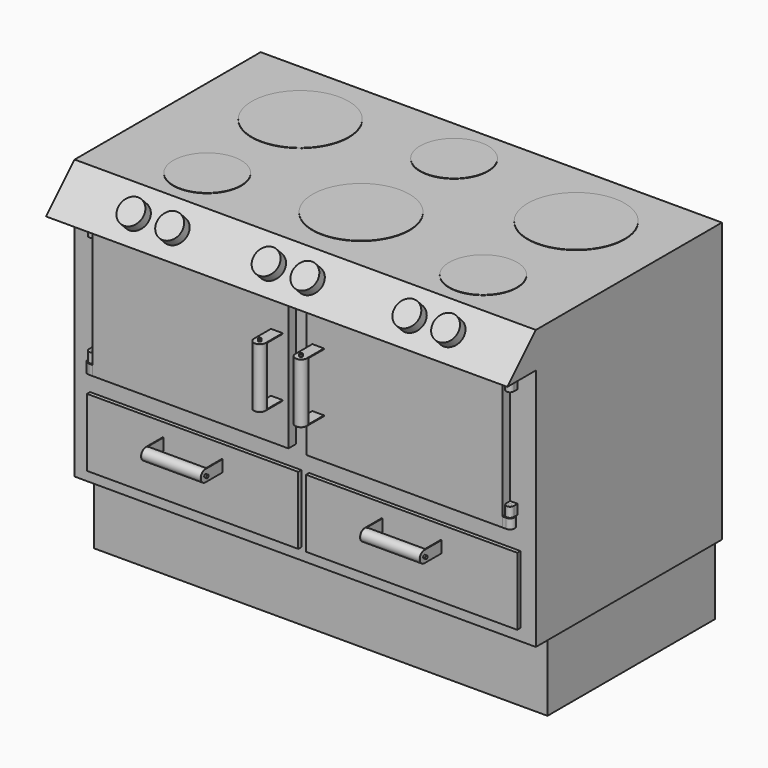
from build123d import *

# Parameters (mm, degrees)
F5_W           = 1190
F5_H           = 600
F6_DEPTH       = 720
F7_T           = -5
F8_W           = 465
F8_H           = 320
F9_DEPTH       = 25
F10_W          = 475
F10_H          = 330
F10_W_2        = 465
F10_H_2        = 320
F11_DEPTH      = 415
F12_W          = 475
F12_H          = 330
F13_DEPTH      = 5
F14_W          = 505
F14_H          = 150
F15_DEPTH      = 25
F16_W          = 515
F16_H          = 160
F16_W_2        = 505
F16_H_2        = 150
F17_DEPTH      = 470
F18_W          = 515
F18_H          = 160
F19_DEPTH      = 5
F20_R          = 6
F21_DEPTH      = 10
F22_R          = 6
F23_DEPTH      = 180
F25_DEPTH      = 10
F27_DEPTH      = 180
F28_W          = 505
F28_H          = 150
F29_DEPTH      = 475
F30_T          = -1
F30_2_T        = -1
F31_W          = 545
F31_H          = 175
F32_DEPTH      = 10
F33_W          = 505
F33_H          = 360
F34_DEPTH      = 25
F36_DEPTH      = 1190
F37_R          = 87.5
F38_DEPTH      = 1
F37_R_2        = 125
F39_R          = 4
F40_DEPTH      = 25
F41_R          = 4
F42_DEPTH      = 25
F43_R          = 4
F44_DEPTH      = 50
F49_R          = 45
F49_R_2        = 15
F50_DEPTH      = 25
F52_DEPTH      = 40
F54_R          = 4
F55_DEPTH      = 100
F56_W          = 475
F56_H          = 330
F56_W_2        = 471
F56_H_2        = 326
F57_DEPTH      = 80
F58_W          = 475
F58_H          = 330
F59_DEPTH      = 2
F60_W          = 475
F60_H          = 330
F61_DEPTH      = 502
F62_R          = 15
F62_R_2        = 4
F63_DEPTH      = 75
F64_R          = 4
F65_DEPTH      = 2
F67_R          = 4
F68_DEPTH      = 5
F68_DEPTH_BACK = 159
F71_R          = 15
F71_R_2        = 4
F72_DEPTH      = 75
F73_R          = 4
F74_DEPTH      = 2
F76_R          = 4
F77_DEPTH      = 5
F77_DEPTH_BACK = 159
F79_R          = 32.5
F80_DEPTH      = 25


with BuildPart() as f6:
    # F5 (on offset) → F6 (new body)
    with BuildSketch(Plane.XY.offset(190)):
        with Locations((595, -300)):
            Rectangle(F5_W, F5_H)
    extrude(amount=F6_DEPTH)

    # F7
    f7_openings = [f6.faces().sort_by_distance(p)[0] for p in [
        (595, 0, 550),
    ]]
    offset(amount=F7_T, openings=f7_openings)

    # F8 (on face) → F9 (cut)
    with BuildSketch(Plane.XZ.offset(600)):
        with Locations((870.8333333333, 630)):
            Rectangle(F8_W, F8_H)
        with Locations((319.1666666667, 630)):
            Rectangle(F8_W, F8_H)
    extrude(amount=-F9_DEPTH, mode=Mode.SUBTRACT)

    # F10 (on face) → F11 (join)
    with BuildSketch(Plane(origin=(0, -595, 0), x_dir=(-1, 0, 0), z_dir=(0, 1, 0))):
        with Locations((-870.8333333333, 630)):
            Rectangle(F10_W, F10_H)
        with Locations((-870.8333333333, 630)):
            Rectangle(F10_W_2, F10_H_2, mode=Mode.SUBTRACT)
        with Locations((-319.1666666667, 630)):
            Rectangle(F10_W, F10_H)
        with Locations((-319.1666666667, 630)):
            Rectangle(F10_W_2, F10_H_2, mode=Mode.SUBTRACT)
    extrude(amount=F11_DEPTH)

    # F12 (on face) → F13 (join)
    with BuildSketch(Plane(origin=(0, -180, 0), x_dir=(-1, 0, 0), z_dir=(0, 1, 0))):
        with Locations((-870.8333333333, 630)):
            Rectangle(F12_W, F12_H)
        with Locations((-319.1666666667, 630)):
            Rectangle(F12_W, F12_H)
    extrude(amount=F13_DEPTH)

    # F14 (on face) → F15 (cut)
    with BuildSketch(Plane.XZ.offset(600)):
        with Locations((312.5, 315)):
            Rectangle(F14_W, F14_H)
        with Locations((877.5, 315)):
            Rectangle(F14_W, F14_H)
    extrude(amount=-F15_DEPTH, mode=Mode.SUBTRACT)

    # F16 (on face) → F17 (join)
    with BuildSketch(Plane(origin=(0, -595, 0), x_dir=(-1, 0, 0), z_dir=(0, 1, 0))):
        with Locations((-877.5, 315)):
            Rectangle(F16_W, F16_H)
        with Locations((-877.5, 315)):
            Rectangle(F16_W_2, F16_H_2, mode=Mode.SUBTRACT)
        with Locations((-312.5, 315)):
            Rectangle(F16_W, F16_H)
        with Locations((-312.5, 315)):
            Rectangle(F16_W_2, F16_H_2, mode=Mode.SUBTRACT)
    extrude(amount=F17_DEPTH)

    # F18 (on face) → F19 (join)
    with BuildSketch(Plane(origin=(0, -125, 0), x_dir=(-1, 0, 0), z_dir=(0, 1, 0))):
        with Locations((-877.5, 315)):
            Rectangle(F18_W, F18_H)
        with Locations((-312.5, 315)):
            Rectangle(F18_W, F18_H)
    extrude(amount=F19_DEPTH)

    # F35 (on face) → F36 (join, through all)
    with BuildSketch(Plane(origin=(0, 0, 0), x_dir=(0, -1, 0), z_dir=(-1, 0, 0))):
        Polygon((691.9238815543, 818.0761184457), (600, 910), (600, 818.0761184457), align=None)
    extrude(amount=-F36_DEPTH)

    # F49 (on face) → F50 (cut)
    with BuildSketch(Plane(origin=(0, -175, 0), x_dir=(-1, 0, 0), z_dir=(0, 1, 0))):
        with Locations((-870.8333333333, 630)):
            Circle(F49_R)
        with Locations((-1058.3333333333, 745)):
            Circle(F49_R_2)
        with Locations((-1058.3333333333, 630)):
            Circle(F49_R_2)
        with Locations((-1058.3333333333, 515)):
            Circle(F49_R_2)
        with Locations((-691.8123364449, 745)):
            Circle(F49_R_2)
        with Locations((-691.8123364449, 630)):
            Circle(F49_R_2)
        with Locations((-683.3333333333, 515)):
            Circle(F49_R_2)
        with Locations((-319.1666666667, 630)):
            Circle(F49_R)
        with Locations((-506.6666666667, 745)):
            Circle(F49_R_2)
        with Locations((-506.6666666667, 630)):
            Circle(F49_R_2)
        with Locations((-506.6666666667, 515)):
            Circle(F49_R_2)
        with Locations((-131.6666666667, 630)):
            Circle(F49_R_2)
        with Locations((-131.6666666667, 745)):
            Circle(F49_R_2)
        with Locations((-131.6666666667, 515)):
            Circle(F49_R_2)
        with Locations((-319.1666666667, 515)):
            Circle(F49_R_2)
        with Locations((-319.1666666667, 745)):
            Circle(F49_R_2)
        with Locations((-870.8333333333, 745)):
            Circle(F49_R_2)
        with Locations((-870.8333333333, 515)):
            Circle(F49_R_2)
    extrude(amount=-F50_DEPTH, mode=Mode.SUBTRACT)


with BuildPart() as f21:
    # F20 (on face) → F21 (new body)
    with BuildSketch(Plane(origin=(0, 0, 190), x_dir=(1, 0, 0), z_dir=(0, 0, -1))):
        Polygon((44.5151724427, 490.5), (55.4848275573, 490.5), (60.9696551146, 500), (55.4848275573, 509.5), (44.5151724427, 509.5), (39.0303448854, 500), align=None)
        with Locations((50, 500)):
            Circle(F20_R, mode=Mode.SUBTRACT)
    extrude(amount=F21_DEPTH)


with BuildPart() as f21b:
    # F20 (on face) → F21, piece 2 (new body)
    with BuildSketch(Plane(origin=(0, 0, 190), x_dir=(1, 0, 0), z_dir=(0, 0, -1))):
        Polygon((1134.5151724427, 490.5), (1145.4848275573, 490.5), (1150.9696551146, 500), (1145.4848275573, 509.5), (1134.5151724427, 509.5), (1129.0303448854, 500), align=None)
        with Locations((1140, 500)):
            Circle(F20_R, mode=Mode.SUBTRACT)
    extrude(amount=F21_DEPTH)


with BuildPart() as f21c:
    # F20 (on face) → F21, piece 3 (new body)
    with BuildSketch(Plane(origin=(0, 0, 190), x_dir=(1, 0, 0), z_dir=(0, 0, -1))):
        Polygon((1145.4848275573, 40.5), (1150.9696551146, 50), (1145.4848275573, 59.5), (1134.5151724427, 59.5), (1129.0303448854, 50), (1134.5151724427, 40.5), align=None)
        with Locations((1140, 50)):
            Circle(F20_R, mode=Mode.SUBTRACT)
    extrude(amount=F21_DEPTH)


with BuildPart() as f21d:
    # F20 (on face) → F21, piece 4 (new body)
    with BuildSketch(Plane(origin=(0, 0, 190), x_dir=(1, 0, 0), z_dir=(0, 0, -1))):
        Polygon((40.0368294952, 45.4099491479), (48.9935153902, 39.0766158145), (58.956685895, 43.6666666667), (59.9631705048, 54.5900508521), (51.0064846098, 60.9233841855), (41.043314105, 56.3333333333), align=None)
        with Locations((50, 50)):
            Circle(F20_R, mode=Mode.SUBTRACT)
    extrude(amount=F21_DEPTH)


with BuildPart() as f23:
    # F22 (on face) → F23 (new body)
    with BuildSketch(Plane(origin=(0, 0, 190), x_dir=(1, 0, 0), z_dir=(0, 0, -1))):
        with Locations((50, 500)):
            Circle(F22_R)
    extrude(amount=F23_DEPTH)

    # F24 (on face) → F25, piece 4 (join)
    with BuildSketch(Plane(origin=(0, 0, 10), x_dir=(1, 0, 0), z_dir=(0, 0, -1))):
        Polygon((44.5151724427, 490.5), (55.4848275573, 490.5), (60.9696551146, 500), (55.4848275573, 509.5), (44.5151724427, 509.5), (39.0303448854, 500), align=None)
    extrude(amount=F25_DEPTH)


with BuildPart() as f23b:
    # F22 (on face) → F23, piece 2 (new body)
    with BuildSketch(Plane(origin=(0, 0, 190), x_dir=(1, 0, 0), z_dir=(0, 0, -1))):
        with Locations((50, 50)):
            Circle(F22_R)
    extrude(amount=F23_DEPTH)

    # F24 (on face) → F25, piece 3 (join)
    with BuildSketch(Plane(origin=(0, 0, 10), x_dir=(1, 0, 0), z_dir=(0, 0, -1))):
        Polygon((59.5, 44.5151724427), (59.5, 55.4848275573), (50, 60.9696551146), (40.5, 55.4848275573), (40.5, 44.5151724427), (50, 39.0303448854), align=None)
    extrude(amount=F25_DEPTH)


with BuildPart() as f23c:
    # F22 (on face) → F23, piece 3 (new body)
    with BuildSketch(Plane(origin=(0, 0, 190), x_dir=(1, 0, 0), z_dir=(0, 0, -1))):
        with Locations((1140, 50)):
            Circle(F22_R)
    extrude(amount=F23_DEPTH)

    # F24 (on face) → F25, piece 2 (join)
    with BuildSketch(Plane(origin=(0, 0, 10), x_dir=(1, 0, 0), z_dir=(0, 0, -1))):
        Polygon((1150.278965993, 53.830951768), (1141.8217814447, 60.8173215585), (1131.5428154518, 56.9863697906), (1129.721034007, 46.169048232), (1138.1782185553, 39.1826784415), (1148.4571845482, 43.0136302094), align=None)
    extrude(amount=F25_DEPTH)


with BuildPart() as f23d:
    # F22 (on face) → F23, piece 4 (new body)
    with BuildSketch(Plane(origin=(0, 0, 190), x_dir=(1, 0, 0), z_dir=(0, 0, -1))):
        with Locations((1140, 500)):
            Circle(F22_R)
    extrude(amount=F23_DEPTH)

    # F24 (on face) → F25 (join)
    with BuildSketch(Plane(origin=(0, 0, 10), x_dir=(1, 0, 0), z_dir=(0, 0, -1))):
        Polygon((1141.8217814447, 489.1826784415), (1150.278965993, 496.169048232), (1148.4571845482, 506.9863697906), (1138.1782185553, 510.8173215585), (1129.721034007, 503.830951768), (1131.5428154518, 493.0136302094), align=None)
    extrude(amount=F25_DEPTH)


with BuildPart() as f27:
    # F26 (on face) → F27 (new body)
    with BuildSketch(Plane(origin=(0, 0, 190), x_dir=(1, 0, 0), z_dir=(0, 0, -1))):
        Polygon((10, 550), (10, 10), (11, 10), (11, 549), (1179, 549), (1179, 10), (1180, 10), (1180, 550), align=None)
    extrude(amount=F27_DEPTH)


with BuildPart() as f29:
    # F28 (on face) → F29 (new body, through all)
    with BuildSketch(Plane.XZ.offset(125)):
        with Locations((312.5, 315)):
            Rectangle(F28_W, F28_H)
    extrude(amount=F29_DEPTH)

    # F30
    f30_openings = [f29.faces().sort_by_distance(p)[0] for p in [
        (312.5, -362.5, 390),
    ]]
    offset(amount=F30_T, openings=f30_openings)

    # F31 (on face) → F32 (join)
    with BuildSketch(Plane.XZ.offset(600)):
        with Locations((312.5, 307.5)):
            Rectangle(F31_W, F31_H)
    extrude(amount=F32_DEPTH)


with BuildPart() as f29b:
    # F28 (on face) → F29, piece 2 (new body, through all)
    with BuildSketch(Plane.XZ.offset(125)):
        with Locations((877.5, 315)):
            Rectangle(F28_W, F28_H)
    extrude(amount=F29_DEPTH)

    # F30#2
    f30_2_openings = [f29b.faces().sort_by_distance(p)[0] for p in [
        (877.5, -362.5, 390),
    ]]
    offset(amount=F30_2_T, openings=f30_2_openings)

    # F31 (on face) → F32, piece 2 (join)
    with BuildSketch(Plane.XZ.offset(600)):
        with Locations((877.5, 307.5)):
            Rectangle(F31_W, F31_H)
    extrude(amount=F32_DEPTH)


with BuildPart() as f34:
    # F33 (on face) → F34 (new body)
    with BuildSketch(Plane.XZ.offset(600)):
        with Locations((319.1666666667, 630)):
            Rectangle(F33_W, F33_H)
    extrude(amount=F34_DEPTH)


with BuildPart() as f34b:
    # F33 (on face) → F34, piece 2 (new body)
    with BuildSketch(Plane.XZ.offset(600)):
        with Locations((870.8333333333, 630)):
            Rectangle(F33_W, F33_H)
    extrude(amount=F34_DEPTH)


with BuildPart() as f38:
    # F37 (on face) → F38 (new body)
    with BuildSketch(Plane.XY.offset(910)):
        with Locations((246.2166398764, -480)):
            Circle(F37_R)
    extrude(amount=F38_DEPTH)


with BuildPart() as f38b:
    # F37 (on face) → F38, piece 2 (new body)
    with BuildSketch(Plane.XY.offset(910)):
        with Locations((246.2166398764, -180)):
            Circle(F37_R_2)
    extrude(amount=F38_DEPTH)


with BuildPart() as f38c:
    # F37 (on face) → F38, piece 3 (new body)
    with BuildSketch(Plane.XY.offset(910)):
        with Locations((595, -420)):
            Circle(F37_R_2)
    extrude(amount=F38_DEPTH)


with BuildPart() as f38d:
    # F37 (on face) → F38, piece 4 (new body)
    with BuildSketch(Plane.XY.offset(910)):
        with Locations((595, -120)):
            Circle(F37_R)
    extrude(amount=F38_DEPTH)


with BuildPart() as f38e:
    # F37 (on face) → F38, piece 5 (new body)
    with BuildSketch(Plane.XY.offset(910)):
        with Locations((958.0140978497, -180)):
            Circle(F37_R_2)
    extrude(amount=F38_DEPTH)


with BuildPart() as f38f:
    # F37 (on face) → F38, piece 6 (new body)
    with BuildSketch(Plane.XY.offset(910)):
        with Locations((958.0140978497, -480)):
            Circle(F37_R)
    extrude(amount=F38_DEPTH)


with BuildPart() as f40:
    # F39 (on face) → F40 (new body)
    with BuildSketch(Plane(origin=(0, 0, 450), x_dir=(1, 0, 0), z_dir=(0, 0, -1))):
        with BuildLine():
            Line((66.6666666667, 600), (66.6666666667, 625))
            Line((66.6666666667, 625), (56.6666666667, 625))
            ThreePointArc((56.6666666667, 625), (44.1666666667, 612.5), (56.6666666667, 600))
            Line((56.6666666667, 600), (66.6666666667, 600))
        make_face()
        with Locations((56.6666666667, 612.5)):
            Circle(F39_R, mode=Mode.SUBTRACT)
    extrude(amount=-F40_DEPTH)


with BuildPart() as f42:
    # F41 (on face) → F42 (new body)
    with BuildSketch(Plane.XY.offset(475)):
        with BuildLine():
            ThreePointArc((47.0310214774, -612.5), (56.6666666667, -622.1356451893), (66.3023118559, -612.5))
            Line((66.3023118559, -612.5), (66.3023118559, -600))
            Line((66.3023118559, -600), (47.0310214774, -600))
            Line((47.0310214774, -600), (47.0310214774, -612.5))
        make_face()
        with Locations((56.6666666667, -612.5)):
            Circle(F41_R, mode=Mode.SUBTRACT)
    extrude(amount=F42_DEPTH)


with BuildPart() as f44:
    # F43 (on face) → F44 (new body, through all)
    with BuildSketch(Plane.XY.offset(500)):
        with Locations((56.6666666667, -612.5)):
            Circle(F43_R)
    extrude(amount=-F44_DEPTH)


with BuildPart() as f46_1:
    # F46: instance of F40
    add(f40.part.mirror(Plane(origin=(319.1666666667, -612.5, 630), x_dir=(1, 0, 0), z_dir=(0, 0, 1))))


with BuildPart() as f46_2:
    # F46: instance of F42
    add(f42.part.mirror(Plane(origin=(319.1666666667, -612.5, 630), x_dir=(1, 0, 0), z_dir=(0, 0, 1))))


with BuildPart() as f46_3:
    # F46: instance of F44
    add(f44.part.mirror(Plane(origin=(319.1666666667, -612.5, 630), x_dir=(1, 0, 0), z_dir=(0, 0, 1))))


with BuildPart() as f48_1:
    # F48: instance of F46_1
    add(f46_1.part.mirror(Plane(origin=(595, -612.5, 630), x_dir=(0, 1, 0), z_dir=(1, 0, 0))))


with BuildPart() as f48_2:
    # F48: instance of F40
    add(f40.part.mirror(Plane(origin=(595, -612.5, 630), x_dir=(0, 1, 0), z_dir=(1, 0, 0))))


with BuildPart() as f48_3:
    # F48: instance of F46_2
    add(f46_2.part.mirror(Plane(origin=(595, -612.5, 630), x_dir=(0, 1, 0), z_dir=(1, 0, 0))))


with BuildPart() as f48_4:
    # F48: instance of F46_3
    add(f46_3.part.mirror(Plane(origin=(595, -612.5, 630), x_dir=(0, 1, 0), z_dir=(1, 0, 0))))


with BuildPart() as f48_5:
    # F48: instance of F42
    add(f42.part.mirror(Plane(origin=(595, -612.5, 630), x_dir=(0, 1, 0), z_dir=(1, 0, 0))))


with BuildPart() as f48_6:
    # F48: instance of F44
    add(f44.part.mirror(Plane(origin=(595, -612.5, 630), x_dir=(0, 1, 0), z_dir=(1, 0, 0))))


with BuildPart() as f52:
    # F51 (on face) → F52 (new body)
    with BuildSketch(Plane(origin=(0, -175, 0), x_dir=(-1, 0, 0), z_dir=(0, 1, 0))):
        with BuildLine():
            ThreePointArc((-849.5774378599, 629.5), (-849.5730279796, 629.7499827139), (-849.5715579518, 630))
            ThreePointArc((-849.5715579518, 630), (-849.5730279796, 630.2500172861), (-849.5774378599, 630.5))
            Line((-849.5774378599, 630.5), (-850.8333333333, 630.5))
            Line((-850.8333333333, 630.5), (-850.8333333333, 629.5))
            Line((-850.8333333333, 629.5), (-849.5774378599, 629.5))
        make_face()
        with BuildLine():
            ThreePointArc((-849.5774378599, 630.5), (-849.5730279796, 630.2500172861), (-849.5715579518, 630))
            ThreePointArc((-849.5715579518, 630), (-849.5730279796, 629.7499827139), (-849.5774378599, 629.5))
            Line((-849.5774378599, 629.5), (-800.8333333333, 629.5))
            Line((-800.8333333333, 629.5), (-800.8333333333, 630.5))
            Line((-800.8333333333, 630.5), (-849.5774378599, 630.5))
        make_face()
        with BuildLine():
            Line((-850.8333333333, 630.5), (-849.5774378599, 630.5))
            ThreePointArc((-849.5774378599, 630.5), (-849.8333256886, 633.3260744576), (-850.4632669365, 636.0929046738))
            Line((-850.4632669365, 636.0929046738), (-851.6576945102, 635.7048116294))
            Line((-851.6576945102, 635.7048116294), (-851.9667115046, 636.6558681456))
            Line((-851.9667115046, 636.6558681456), (-850.7722839308, 637.0439611901))
            ThreePointArc((-850.7722839308, 637.0439611901), (-851.8889527525, 639.6526440308), (-853.3430600385, 642.0893933864))
            Line((-853.3430600385, 642.0893933864), (-854.3591008197, 641.3511965487))
            Line((-854.3591008197, 641.3511965487), (-854.946886072, 642.160213543))
            Line((-854.946886072, 642.160213543), (-853.9308452908, 642.8984103807))
            ThreePointArc((-853.9308452908, 642.8984103807), (-855.798987781, 645.0343455524), (-857.9349229526, 646.9024880425))
            Line((-857.9349229526, 646.9024880425), (-858.6731197903, 645.8864472614))
            Line((-858.6731197903, 645.8864472614), (-859.4821367847, 646.4742325136))
            Line((-859.4821367847, 646.4742325136), (-858.743939947, 647.4902732948))
            ThreePointArc((-858.743939947, 647.4902732948), (-861.1806893025, 648.9443805808), (-863.7893721432, 650.0610494025))
            Line((-863.7893721432, 650.0610494025), (-864.1774651877, 648.8666218287))
            Line((-864.1774651877, 648.8666218287), (-865.128521704, 649.1756388231))
            Line((-865.128521704, 649.1756388231), (-864.7404286595, 650.3700663969))
            ThreePointArc((-864.7404286595, 650.3700663969), (-867.5072588757, 651.0000076447), (-870.3333333333, 651.2558954734))
            Line((-870.3333333333, 651.2558954734), (-870.3333333333, 650))
            Line((-870.3333333333, 650), (-871.3333333333, 650))
            Line((-871.3333333333, 650), (-871.3333333333, 651.2558954734))
            ThreePointArc((-871.3333333333, 651.2558954734), (-874.159407791, 651.0000076447), (-876.9262380071, 650.3700663969))
            Line((-876.9262380071, 650.3700663969), (-876.5381449627, 649.1756388231))
            Line((-876.5381449627, 649.1756388231), (-877.489201479, 648.8666218287))
            Line((-877.489201479, 648.8666218287), (-877.8772945234, 650.0610494025))
            ThreePointArc((-877.8772945234, 650.0610494025), (-880.4859773642, 648.9443805808), (-882.9227267197, 647.4902732948))
            Line((-882.9227267197, 647.4902732948), (-882.184529882, 646.4742325136))
            Line((-882.184529882, 646.4742325136), (-882.9935468764, 645.8864472614))
            Line((-882.9935468764, 645.8864472614), (-883.7317437141, 646.9024880425))
            ThreePointArc((-883.7317437141, 646.9024880425), (-885.8676788857, 645.0343455524), (-887.7358213758, 642.8984103807))
            Line((-887.7358213758, 642.8984103807), (-886.7197805947, 642.160213543))
            Line((-886.7197805947, 642.160213543), (-887.307565847, 641.3511965487))
            Line((-887.307565847, 641.3511965487), (-888.3236066281, 642.0893933864))
            ThreePointArc((-888.3236066281, 642.0893933864), (-889.7777139141, 639.6526440308), (-890.8943827358, 637.0439611901))
            Line((-890.8943827358, 637.0439611901), (-889.699955162, 636.6558681456))
            Line((-889.699955162, 636.6558681456), (-890.0089721564, 635.7048116293))
            Line((-890.0089721564, 635.7048116294), (-891.2033997302, 636.0929046738))
            ThreePointArc((-891.2033997302, 636.0929046738), (-891.8333409781, 633.3260744576), (-892.0892288067, 630.5))
            Line((-892.0892288067, 630.5), (-890.8333333333, 630.5))
            Line((-890.8333333333, 630.5), (-890.8333333333, 629.5))
            Line((-890.8333333333, 629.5), (-892.0892288067, 629.5))
            ThreePointArc((-892.0892288067, 629.5), (-891.8333409781, 626.6739255424), (-891.2033997302, 623.9070953262))
            Line((-891.2033997302, 623.9070953262), (-890.0089721564, 624.2951883706))
            Line((-890.0089721564, 624.2951883706), (-889.699955162, 623.3441318544))
            Line((-889.699955162, 623.3441318544), (-890.8943827358, 622.9560388099))
            ThreePointArc((-890.8943827358, 622.9560388099), (-889.7777139141, 620.3473559692), (-888.3236066281, 617.9106066136))
            Line((-888.3236066281, 617.9106066136), (-887.307565847, 618.6488034513))
            Line((-887.307565847, 618.6488034513), (-886.7197805947, 617.839786457))
            Line((-886.7197805947, 617.839786457), (-887.7358213758, 617.1015896193))
            ThreePointArc((-887.7358213758, 617.1015896193), (-885.8676788857, 614.9656544476), (-883.7317437141, 613.0975119575))
            Line((-883.7317437141, 613.0975119575), (-882.9935468764, 614.1135527386))
            Line((-882.9935468764, 614.1135527386), (-882.184529882, 613.5257674864))
            Line((-882.184529882, 613.5257674864), (-882.9227267197, 612.5097267052))
            ThreePointArc((-882.9227267197, 612.5097267052), (-880.4859773642, 611.0556194192), (-877.8772945234, 609.9389505975))
            Line((-877.8772945234, 609.9389505975), (-877.489201479, 611.1333781713))
            Line((-877.489201479, 611.1333781713), (-876.5381449627, 610.8243611769))
            Line((-876.5381449627, 610.8243611769), (-876.9262380071, 609.6299336031))
            ThreePointArc((-876.9262380071, 609.6299336031), (-874.159407791, 608.9999923553), (-871.3333333333, 608.7441045266))
            Line((-871.3333333333, 608.7441045266), (-871.3333333333, 610))
            Line((-871.3333333333, 610), (-870.3333333333, 610))
            Line((-870.3333333333, 610), (-870.3333333333, 608.7441045266))
            ThreePointArc((-870.3333333333, 608.7441045266), (-867.5072588757, 608.9999923553), (-864.7404286595, 609.6299336031))
            Line((-864.7404286595, 609.6299336031), (-865.128521704, 610.8243611769))
            Line((-865.128521704, 610.8243611769), (-864.1774651877, 611.1333781713))
            Line((-864.1774651877, 611.1333781713), (-863.7893721432, 609.9389505975))
            ThreePointArc((-863.7893721432, 609.9389505975), (-861.1806893025, 611.0556194192), (-858.743939947, 612.5097267052))
            Line((-858.743939947, 612.5097267052), (-859.4821367847, 613.5257674864))
            Line((-859.4821367847, 613.5257674864), (-858.6731197903, 614.1135527386))
            Line((-858.6731197903, 614.1135527386), (-857.9349229526, 613.0975119575))
            ThreePointArc((-857.9349229526, 613.0975119575), (-855.798987781, 614.9656544476), (-853.9308452908, 617.1015896193))
            Line((-853.9308452908, 617.1015896193), (-854.946886072, 617.839786457))
            Line((-854.946886072, 617.839786457), (-854.3591008197, 618.6488034513))
            Line((-854.3591008197, 618.6488034513), (-853.3430600385, 617.9106066136))
            ThreePointArc((-853.3430600385, 617.9106066136), (-851.8889527525, 620.3473559692), (-850.7722839308, 622.9560388099))
            Line((-850.7722839308, 622.9560388099), (-851.9667115046, 623.3441318544))
            Line((-851.9667115046, 623.3441318544), (-851.6576945102, 624.2951883707))
            Line((-851.6576945102, 624.2951883706), (-850.4632669365, 623.9070953262))
            ThreePointArc((-850.4632669365, 623.9070953262), (-849.8333256886, 626.6739255424), (-849.5774378599, 629.5))
            Line((-849.5774378599, 629.5), (-850.8333333333, 629.5))
            Line((-850.8333333333, 629.5), (-850.8333333333, 630.5))
        make_face()
        with BuildLine():
            Line((-851.6576945102, 635.7048116294), (-850.4632669365, 636.0929046738))
            ThreePointArc((-850.4632669365, 636.0929046738), (-850.6121833087, 636.5702499235), (-850.7722839308, 637.0439611901))
            Line((-850.7722839308, 637.0439611901), (-851.9667115046, 636.6558681456))
            Line((-851.9667115046, 636.6558681456), (-851.6576945102, 635.7048116294))
        make_face()
        with BuildLine():
            ThreePointArc((-850.7722839308, 637.0439611901), (-850.6121833087, 636.5702499235), (-850.4632669365, 636.0929046738))
            Line((-850.4632669365, 636.0929046738), (-804.1048686955, 651.1556613481))
            Line((-804.1048686955, 651.1556613481), (-804.4138856899, 652.1067178644))
            Line((-804.4138856899, 652.1067178644), (-850.7722839308, 637.0439611901))
        make_face()
        with BuildLine():
            Line((-804.1048686955, 608.8443386519), (-850.4632669365, 623.9070953262))
            ThreePointArc((-850.4632669365, 623.9070953262), (-850.6121833087, 623.4297500765), (-850.7722839308, 622.9560388099))
            Line((-850.7722839308, 622.9560388099), (-804.4138856899, 607.8932821356))
            Line((-804.4138856899, 607.8932821356), (-804.1048686955, 608.8443386519))
        make_face()
        with BuildLine():
            ThreePointArc((-850.7722839308, 622.9560388099), (-850.6121833087, 623.4297500765), (-850.4632669365, 623.9070953262))
            Line((-850.4632669365, 623.9070953262), (-851.6576945102, 624.2951883706))
            Line((-851.6576945102, 624.2951883707), (-851.9667115046, 623.3441318544))
            Line((-851.9667115046, 623.3441318544), (-850.7722839308, 622.9560388099))
        make_face()
        with BuildLine():
            Line((-854.3591008197, 641.3511965487), (-853.3430600385, 642.0893933864))
            ThreePointArc((-853.3430600385, 642.0893933864), (-853.6321957191, 642.4973580068), (-853.9308452908, 642.8984103807))
            Line((-853.9308452908, 642.8984103807), (-854.946886072, 642.160213543))
            Line((-854.946886072, 642.160213543), (-854.3591008197, 641.3511965487))
        make_face()
        with BuildLine():
            ThreePointArc((-853.9308452908, 642.8984103807), (-853.6321957191, 642.4973580068), (-853.3430600385, 642.0893933864))
            Line((-853.3430600385, 642.0893933864), (-813.9082511009, 670.7404591633))
            Line((-813.9082511009, 670.7404591633), (-814.4960363532, 671.5494761577))
            Line((-814.4960363532, 671.5494761577), (-853.9308452908, 642.8984103807))
        make_face()
        with BuildLine():
            Line((-813.9082511009, 589.2595408367), (-853.3430600385, 617.9106066136))
            ThreePointArc((-853.3430600385, 617.9106066136), (-853.6321957191, 617.5026419932), (-853.9308452908, 617.1015896193))
            Line((-853.9308452908, 617.1015896193), (-814.4960363532, 588.4505238423))
            Line((-814.4960363532, 588.4505238423), (-813.9082511009, 589.2595408367))
        make_face()
        with BuildLine():
            ThreePointArc((-853.9308452908, 617.1015896193), (-853.6321957191, 617.5026419932), (-853.3430600385, 617.9106066136))
            Line((-853.3430600385, 617.9106066136), (-854.3591008197, 618.6488034513))
            Line((-854.3591008197, 618.6488034513), (-854.946886072, 617.839786457))
            Line((-854.946886072, 617.839786457), (-853.9308452908, 617.1015896193))
        make_face()
        with BuildLine():
            Line((-858.6731197903, 645.8864472614), (-857.9349229526, 646.9024880425))
            ThreePointArc((-857.9349229526, 646.9024880425), (-858.3359753265, 647.2011376143), (-858.743939947, 647.4902732948))
            Line((-858.743939947, 647.4902732948), (-859.4821367847, 646.4742325136))
            Line((-859.4821367847, 646.4742325136), (-858.6731197903, 645.8864472614))
        make_face()
        with BuildLine():
            ThreePointArc((-858.743939947, 647.4902732948), (-858.3359753265, 647.2011376143), (-857.9349229526, 646.9024880425))
            Line((-857.9349229526, 646.9024880425), (-829.2838571757, 686.3372969801))
            Line((-829.2838571757, 686.3372969801), (-830.09287417, 686.9250822324))
            Line((-830.09287417, 686.9250822324), (-858.743939947, 647.4902732948))
        make_face()
        with BuildLine():
            Line((-829.2838571757, 573.6627030199), (-857.9349229526, 613.0975119575))
            ThreePointArc((-857.9349229526, 613.0975119575), (-858.3359753265, 612.7988623857), (-858.743939947, 612.5097267052))
            Line((-858.743939947, 612.5097267052), (-830.09287417, 573.0749177676))
            Line((-830.09287417, 573.0749177676), (-829.2838571757, 573.6627030199))
        make_face()
        with BuildLine():
            ThreePointArc((-858.743939947, 612.5097267052), (-858.3359753265, 612.7988623857), (-857.9349229526, 613.0975119575))
            Line((-857.9349229526, 613.0975119575), (-858.6731197903, 614.1135527386))
            Line((-858.6731197903, 614.1135527386), (-859.4821367847, 613.5257674864))
            Line((-859.4821367847, 613.5257674864), (-858.743939947, 612.5097267052))
        make_face()
        with BuildLine():
            Line((-864.1774651877, 648.8666218287), (-863.7893721432, 650.0610494025))
            ThreePointArc((-863.7893721432, 650.0610494025), (-864.2630834098, 650.2211500247), (-864.7404286595, 650.3700663969))
            Line((-864.7404286595, 650.3700663969), (-865.128521704, 649.1756388231))
            Line((-865.128521704, 649.1756388231), (-864.1774651877, 648.8666218287))
        make_face()
        with BuildLine():
            ThreePointArc((-864.7404286595, 650.3700663969), (-864.2630834098, 650.2211500247), (-863.7893721432, 650.0610494025))
            Line((-863.7893721432, 650.0610494025), (-848.7266154689, 696.4194476435))
            Line((-848.7266154689, 696.4194476435), (-849.6776719852, 696.7284646378))
            Line((-849.6776719852, 696.7284646378), (-864.7404286595, 650.3700663969))
        make_face()
        with BuildLine():
            Line((-848.7266154689, 563.5805523565), (-863.7893721432, 609.9389505975))
            ThreePointArc((-863.7893721432, 609.9389505975), (-864.2630834098, 609.7788499753), (-864.7404286595, 609.6299336031))
            Line((-864.7404286595, 609.6299336031), (-849.6776719852, 563.2715353622))
            Line((-849.6776719852, 563.2715353622), (-848.7266154689, 563.5805523565))
        make_face()
        with BuildLine():
            ThreePointArc((-864.7404286595, 609.6299336031), (-864.2630834098, 609.7788499753), (-863.7893721432, 609.9389505975))
            Line((-863.7893721432, 609.9389505975), (-864.1774651877, 611.1333781713))
            Line((-864.1774651877, 611.1333781713), (-865.128521704, 610.8243611769))
            Line((-865.128521704, 610.8243611769), (-864.7404286595, 609.6299336031))
        make_face()
        with BuildLine():
            Line((-870.3333333333, 650), (-870.3333333333, 651.2558954734))
            ThreePointArc((-870.3333333333, 651.2558954734), (-870.8333333333, 651.2617753816), (-871.3333333333, 651.2558954734))
            Line((-871.3333333333, 651.2558954734), (-871.3333333333, 650))
            Line((-871.3333333333, 650), (-870.3333333333, 650))
        make_face()
        with BuildLine():
            ThreePointArc((-871.3333333333, 651.2558954734), (-870.8333333333, 651.2617753816), (-870.3333333333, 651.2558954734))
            Line((-870.3333333333, 651.2558954734), (-870.3333333333, 700))
            Line((-870.3333333333, 700), (-871.3333333333, 700))
            Line((-871.3333333333, 700), (-871.3333333333, 651.2558954734))
        make_face()
        with BuildLine():
            Line((-870.3333333333, 560), (-870.3333333333, 608.7441045266))
            ThreePointArc((-870.3333333333, 608.7441045266), (-870.8333333333, 608.7382246184), (-871.3333333333, 608.7441045266))
            Line((-871.3333333333, 608.7441045266), (-871.3333333333, 560))
            Line((-871.3333333333, 560), (-870.3333333333, 560))
        make_face()
        with BuildLine():
            ThreePointArc((-871.3333333333, 608.7441045266), (-870.8333333333, 608.7382246184), (-870.3333333333, 608.7441045266))
            Line((-870.3333333333, 608.7441045266), (-870.3333333333, 610))
            Line((-870.3333333333, 610), (-871.3333333333, 610))
            Line((-871.3333333333, 610), (-871.3333333333, 608.7441045266))
        make_face()
        with BuildLine():
            Line((-876.5381449627, 649.1756388231), (-876.9262380071, 650.3700663969))
            ThreePointArc((-876.9262380071, 650.3700663969), (-877.4035832568, 650.2211500247), (-877.8772945234, 650.0610494025))
            Line((-877.8772945234, 650.0610494025), (-877.489201479, 648.8666218287))
            Line((-877.489201479, 648.8666218287), (-876.5381449627, 649.1756388231))
        make_face()
        with BuildLine():
            ThreePointArc((-877.8772945234, 650.0610494025), (-877.4035832568, 650.2211500247), (-876.9262380071, 650.3700663969))
            Line((-876.9262380071, 650.3700663969), (-891.9889946814, 696.7284646378))
            Line((-891.9889946814, 696.7284646378), (-892.9400511977, 696.4194476435))
            Line((-892.9400511977, 696.4194476435), (-877.8772945234, 650.0610494025))
        make_face()
        with BuildLine():
            Line((-891.9889946814, 563.2715353622), (-876.9262380071, 609.6299336031))
            ThreePointArc((-876.9262380071, 609.6299336031), (-877.4035832568, 609.7788499753), (-877.8772945234, 609.9389505975))
            Line((-877.8772945234, 609.9389505975), (-892.9400511977, 563.5805523565))
            Line((-892.9400511977, 563.5805523565), (-891.9889946814, 563.2715353622))
        make_face()
        with BuildLine():
            ThreePointArc((-877.8772945234, 609.9389505975), (-877.4035832568, 609.7788499753), (-876.9262380071, 609.6299336031))
            Line((-876.9262380071, 609.6299336031), (-876.5381449627, 610.8243611769))
            Line((-876.5381449627, 610.8243611769), (-877.489201479, 611.1333781713))
            Line((-877.489201479, 611.1333781713), (-877.8772945234, 609.9389505975))
        make_face()
        with BuildLine():
            Line((-882.184529882, 646.4742325136), (-882.9227267197, 647.4902732948))
            ThreePointArc((-882.9227267197, 647.4902732948), (-883.3306913402, 647.2011376143), (-883.7317437141, 646.9024880425))
            Line((-883.7317437141, 646.9024880425), (-882.9935468764, 645.8864472614))
            Line((-882.9935468764, 645.8864472614), (-882.184529882, 646.4742325136))
        make_face()
        with BuildLine():
            ThreePointArc((-883.7317437141, 646.9024880425), (-883.3306913402, 647.2011376143), (-882.9227267197, 647.4902732948))
            Line((-882.9227267197, 647.4902732948), (-911.5737924966, 686.9250822324))
            Line((-911.5737924966, 686.9250822324), (-912.382809491, 686.3372969801))
            Line((-912.382809491, 686.3372969801), (-883.7317437141, 646.9024880425))
        make_face()
        with BuildLine():
            Line((-911.5737924966, 573.0749177676), (-882.9227267197, 612.5097267052))
            ThreePointArc((-882.9227267197, 612.5097267052), (-883.3306913402, 612.7988623857), (-883.7317437141, 613.0975119575))
            Line((-883.7317437141, 613.0975119575), (-912.382809491, 573.6627030199))
            Line((-912.382809491, 573.6627030199), (-911.5737924966, 573.0749177676))
        make_face()
        with BuildLine():
            ThreePointArc((-883.7317437141, 613.0975119575), (-883.3306913402, 612.7988623857), (-882.9227267197, 612.5097267052))
            Line((-882.9227267197, 612.5097267052), (-882.184529882, 613.5257674864))
            Line((-882.184529882, 613.5257674864), (-882.9935468764, 614.1135527386))
            Line((-882.9935468764, 614.1135527386), (-883.7317437141, 613.0975119575))
        make_face()
        with BuildLine():
            Line((-886.7197805947, 642.160213543), (-887.7358213758, 642.8984103807))
            ThreePointArc((-887.7358213758, 642.8984103807), (-888.0344709476, 642.4973580068), (-888.3236066281, 642.0893933864))
            Line((-888.3236066281, 642.0893933864), (-887.307565847, 641.3511965487))
            Line((-887.307565847, 641.3511965487), (-886.7197805947, 642.160213543))
        make_face()
        with BuildLine():
            ThreePointArc((-888.3236066281, 642.0893933864), (-888.0344709476, 642.4973580068), (-887.7358213758, 642.8984103807))
            Line((-887.7358213758, 642.8984103807), (-927.1706303134, 671.5494761577))
            Line((-927.1706303134, 671.5494761577), (-927.7584155657, 670.7404591633))
            Line((-927.7584155657, 670.7404591633), (-888.3236066281, 642.0893933864))
        make_face()
        with BuildLine():
            Line((-927.1706303134, 588.4505238423), (-887.7358213758, 617.1015896193))
            ThreePointArc((-887.7358213758, 617.1015896193), (-888.0344709476, 617.5026419932), (-888.3236066281, 617.9106066136))
            Line((-888.3236066281, 617.9106066136), (-927.7584155657, 589.2595408367))
            Line((-927.7584155657, 589.2595408367), (-927.1706303134, 588.4505238423))
        make_face()
        with BuildLine():
            ThreePointArc((-888.3236066281, 617.9106066136), (-888.0344709476, 617.5026419932), (-887.7358213758, 617.1015896193))
            Line((-887.7358213758, 617.1015896193), (-886.7197805947, 617.839786457))
            Line((-886.7197805947, 617.839786457), (-887.307565847, 618.6488034513))
            Line((-887.307565847, 618.6488034513), (-888.3236066281, 617.9106066136))
        make_face()
        with BuildLine():
            Line((-889.699955162, 636.6558681456), (-890.8943827358, 637.0439611901))
            ThreePointArc((-890.8943827358, 637.0439611901), (-891.054483358, 636.5702499235), (-891.2033997302, 636.0929046738))
            Line((-891.2033997302, 636.0929046738), (-890.0089721564, 635.7048116294))
            Line((-890.0089721564, 635.7048116293), (-889.699955162, 636.6558681456))
        make_face()
        with BuildLine():
            ThreePointArc((-891.2033997302, 636.0929046738), (-891.054483358, 636.5702499235), (-890.8943827358, 637.0439611901))
            Line((-890.8943827358, 637.0439611901), (-937.2527809768, 652.1067178644))
            Line((-937.2527809768, 652.1067178644), (-937.5617979712, 651.1556613481))
            Line((-937.5617979712, 651.1556613481), (-891.2033997302, 636.0929046738))
        make_face()
        with BuildLine():
            Line((-937.2527809768, 607.8932821356), (-890.8943827358, 622.9560388099))
            ThreePointArc((-890.8943827358, 622.9560388099), (-891.054483358, 623.4297500765), (-891.2033997302, 623.9070953262))
            Line((-891.2033997302, 623.9070953262), (-937.5617979712, 608.8443386519))
            Line((-937.5617979712, 608.8443386519), (-937.2527809768, 607.8932821356))
        make_face()
        with BuildLine():
            ThreePointArc((-891.2033997302, 623.9070953262), (-891.054483358, 623.4297500765), (-890.8943827358, 622.9560388099))
            Line((-890.8943827358, 622.9560388099), (-889.699955162, 623.3441318544))
            Line((-889.699955162, 623.3441318544), (-890.0089721564, 624.2951883706))
            Line((-890.0089721564, 624.2951883706), (-891.2033997302, 623.9070953262))
        make_face()
        with BuildLine():
            Line((-890.8333333333, 630.5), (-892.0892288067, 630.5))
            ThreePointArc((-892.0892288067, 630.5), (-892.0951087149, 630), (-892.0892288067, 629.5))
            Line((-892.0892288067, 629.5), (-890.8333333333, 629.5))
            Line((-890.8333333333, 629.5), (-890.8333333333, 630.5))
        make_face()
        with BuildLine():
            ThreePointArc((-892.0892288067, 629.5), (-892.0951087149, 630), (-892.0892288067, 630.5))
            Line((-892.0892288067, 630.5), (-940.8333333333, 630.5))
            Line((-940.8333333333, 630.5), (-940.8333333333, 629.5))
            Line((-940.8333333333, 629.5), (-892.0892288067, 629.5))
        make_face()
    extrude(amount=F52_DEPTH)


with BuildPart() as f53_1:
    # F53: instance of F52
    add(f52.part.mirror(Plane(origin=(595, -612.5, 630), x_dir=(0, 1, 0), z_dir=(1, 0, 0))))

    # F54 (on face) → F55, piece 2 (join)
    with BuildSketch(Plane(origin=(0, -135, 0), x_dir=(-1, 0, 0), z_dir=(0, 1, 0))):
        with Locations((-319.1666666667, 630)):
            Circle(F54_R)
    extrude(amount=F55_DEPTH)


with BuildPart() as f52_1:
    add(f52.part)

    # F54 (on face) → F55 (join)
    with BuildSketch(Plane(origin=(0, -135, 0), x_dir=(-1, 0, 0), z_dir=(0, 1, 0))):
        with Locations((-870.8333333333, 630)):
            Circle(F54_R)
    extrude(amount=F55_DEPTH)


with BuildPart() as f57:
    # F56 (on face) → F57 (new body)
    with BuildSketch(Plane(origin=(0, -175, 0), x_dir=(-1, 0, 0), z_dir=(0, 1, 0))):
        with Locations((-870.8333333333, 630)):
            Rectangle(F56_W, F56_H)
        with Locations((-870.8333333333, 630)):
            Rectangle(F56_W_2, F56_H_2, mode=Mode.SUBTRACT)
    extrude(amount=F57_DEPTH)


with BuildPart() as f57b:
    # F56 (on face) → F57, piece 2 (new body)
    with BuildSketch(Plane(origin=(0, -175, 0), x_dir=(-1, 0, 0), z_dir=(0, 1, 0))):
        with Locations((-319.1666666667, 630)):
            Rectangle(F56_W, F56_H)
        with Locations((-319.1666666667, 630)):
            Rectangle(F56_W_2, F56_H_2, mode=Mode.SUBTRACT)
    extrude(amount=F57_DEPTH)


with BuildPart() as f59:
    # F58 (on face) → F59 (new body)
    with BuildSketch(Plane(origin=(0, -95, 0), x_dir=(-1, 0, 0), z_dir=(0, 1, 0))):
        with Locations((-870.8333333333, 630)):
            Rectangle(F58_W, F58_H)
    extrude(amount=F59_DEPTH)


with BuildPart() as f59b:
    # F58 (on face) → F59, piece 2 (new body)
    with BuildSketch(Plane(origin=(0, -95, 0), x_dir=(-1, 0, 0), z_dir=(0, 1, 0))):
        with Locations((-319.1666666667, 630)):
            Rectangle(F58_W, F58_H)
    extrude(amount=F59_DEPTH)


with BuildPart() as f61:
    # F60 (on face) → F61 (new body, through all)
    with BuildSketch(Plane(origin=(0, -595, 0), x_dir=(-1, 0, 0), z_dir=(0, 1, 0))):
        with BuildLine():
            Line((-1103.3333333333, 432), (-638.3333333333, 432))
            ThreePointArc((-638.3333333333, 432), (-611.4632756482, 443.1299423149), (-600.3333333333, 470))
            Line((-600.3333333333, 470), (-600.3333333333, 790))
            ThreePointArc((-600.3333333333, 790), (-611.4632756482, 816.8700576851), (-638.3333333333, 828))
            Line((-638.3333333333, 828), (-1103.3333333333, 828))
            ThreePointArc((-1103.3333333333, 828), (-1130.2033910184, 816.8700576851), (-1141.3333333333, 790))
            Line((-1141.3333333333, 790), (-1141.3333333333, 470))
            ThreePointArc((-1141.3333333333, 470), (-1130.2033910184, 443.1299423149), (-1103.3333333333, 432))
        make_face()
        with Locations((-870.8333333333, 630)):
            Rectangle(F60_W, F60_H, mode=Mode.SUBTRACT)
    extrude(amount=F61_DEPTH)


with BuildPart() as f61b:
    # F60 (on face) → F61, piece 2 (new body, through all)
    with BuildSketch(Plane(origin=(0, -595, 0), x_dir=(-1, 0, 0), z_dir=(0, 1, 0))):
        with BuildLine():
            Line((-551.6666666667, 432), (-86.6666666667, 432))
            ThreePointArc((-86.6666666667, 432), (-59.7966089816, 443.1299423149), (-48.6666666667, 470))
            Line((-48.6666666667, 470), (-48.6666666667, 790))
            ThreePointArc((-48.6666666667, 790), (-59.7966089816, 816.8700576851), (-86.6666666667, 828))
            Line((-86.6666666667, 828), (-551.6666666667, 828))
            ThreePointArc((-551.6666666667, 828), (-578.5367243518, 816.8700576851), (-589.6666666667, 790))
            Line((-589.6666666667, 790), (-589.6666666667, 470))
            ThreePointArc((-589.6666666667, 470), (-578.5367243518, 443.1299423149), (-551.6666666667, 432))
        make_face()
        with Locations((-319.1666666667, 630)):
            Rectangle(F60_W, F60_H, mode=Mode.SUBTRACT)
    extrude(amount=F61_DEPTH)


with BuildPart() as f63:
    # F62 (on mid) → F63 (new body, symmetric)
    with BuildSketch(Plane.XY.offset(630)):
        with Locations((541.6666666667, -680)):
            Circle(F62_R)
        with Locations((541.6666666667, -680)):
            Circle(F62_R_2, mode=Mode.SUBTRACT)
    extrude(amount=F63_DEPTH, both=True)


with BuildPart() as f65:
    # F64 (on face) → F65 (new body)
    with BuildSketch(Plane(origin=(0, 0, 555), x_dir=(1, 0, 0), z_dir=(0, 0, -1))):
        with BuildLine():
            ThreePointArc((556.6666666667, 680), (541.6666666667, 695), (526.6666666667, 680))
            Line((526.6666666667, 680), (526.6666666667, 625))
            Line((526.6666666667, 625), (556.6666666667, 625))
            Line((556.6666666667, 625), (556.6666666667, 680))
        make_face()
        with Locations((541.6666666667, 680)):
            Circle(F64_R, mode=Mode.SUBTRACT)
    extrude(amount=F65_DEPTH)


with BuildPart() as f66_1:
    # F66: instance of F65
    add(f65.part.mirror(Plane(origin=(319.1666666667, -612.5, 630), x_dir=(1, 0, 0), z_dir=(0, 0, 1))))


with BuildPart() as f68:
    # F67 (on face) → F68 (new body, two sides)
    with BuildSketch(Plane(origin=(0, 0, 553), x_dir=(1, 0, 0), z_dir=(0, 0, -1))) as f68_sk:
        with Locations((541.6666666667, 680)):
            Circle(F67_R)
    extrude(amount=F68_DEPTH)
    extrude(f68_sk.sketch, amount=-F68_DEPTH_BACK)


with BuildPart() as f69_1:
    # F69: instance of F65
    add(f65.part.mirror(Plane(origin=(595, -612.5, 630), x_dir=(0, 1, 0), z_dir=(1, 0, 0))))


with BuildPart() as f69_2:
    # F69: instance of F68
    add(f68.part.mirror(Plane(origin=(595, -612.5, 630), x_dir=(0, 1, 0), z_dir=(1, 0, 0))))


with BuildPart() as f69_3:
    # F69: instance of F63
    add(f63.part.mirror(Plane(origin=(595, -612.5, 630), x_dir=(0, 1, 0), z_dir=(1, 0, 0))))


with BuildPart() as f69_4:
    # F69: instance of F66_1
    add(f66_1.part.mirror(Plane(origin=(595, -612.5, 630), x_dir=(0, 1, 0), z_dir=(1, 0, 0))))


with BuildPart() as f72:
    # F71 (on mid) → F72 (new body, symmetric)
    with BuildSketch(Plane.YZ.offset(312.5)):
        with Locations((-665, 345)):
            Circle(F71_R)
        with Locations((-665, 345)):
            Circle(F71_R_2, mode=Mode.SUBTRACT)
    extrude(amount=F72_DEPTH, both=True)


with BuildPart() as f74:
    # F73 (on face) → F74 (new body)
    with BuildSketch(Plane(origin=(237.5, 0, 0), x_dir=(0, -1, 0), z_dir=(-1, 0, 0))):
        with BuildLine():
            ThreePointArc((665, 330), (680, 345), (665, 360))
            Line((665, 360), (610, 360))
            Line((610, 360), (610, 330))
            Line((610, 330), (665, 330))
        make_face()
        with Locations((665, 345)):
            Circle(F73_R, mode=Mode.SUBTRACT)
    extrude(amount=F74_DEPTH)


with BuildPart() as f75_1:
    # F75: instance of F74
    add(f74.part.mirror(Plane(origin=(312.5, -605, 307.5), x_dir=(0, 1, 0), z_dir=(1, 0, 0))))


with BuildPart() as f77:
    # F76 (on face) → F77 (new body, two sides)
    with BuildSketch(Plane(origin=(235.5, 0, 0), x_dir=(0, -1, 0), z_dir=(-1, 0, 0))) as f77_sk:
        with Locations((665, 345)):
            Circle(F76_R)
    extrude(amount=F77_DEPTH)
    extrude(f77_sk.sketch, amount=-F77_DEPTH_BACK)


with BuildPart() as f78_1:
    # F78: instance of F74
    add(f74.part.mirror(Plane(origin=(595, -612.5, 630), x_dir=(0, 1, 0), z_dir=(1, 0, 0))))


with BuildPart() as f78_2:
    # F78: instance of F75_1
    add(f75_1.part.mirror(Plane(origin=(595, -612.5, 630), x_dir=(0, 1, 0), z_dir=(1, 0, 0))))


with BuildPart() as f78_3:
    # F78: instance of F77
    add(f77.part.mirror(Plane(origin=(595, -612.5, 630), x_dir=(0, 1, 0), z_dir=(1, 0, 0))))


with BuildPart() as f78_4:
    # F78: instance of F72
    add(f72.part.mirror(Plane(origin=(595, -612.5, 630), x_dir=(0, 1, 0), z_dir=(1, 0, 0))))


with BuildPart() as f80:
    # F79 (on face) → F80 (new body)
    with BuildSketch(Plane(origin=(0, -755, 755), x_dir=(1, 0, 0), z_dir=(0, -0.7071067812, 0.7071067812))):
        with Locations((196.2166398764, 154.2031021678)):
            Circle(F79_R)
    extrude(amount=F80_DEPTH)


with BuildPart() as f80b:
    # F79 (on face) → F80, piece 2 (new body)
    with BuildSketch(Plane(origin=(0, -755, 755), x_dir=(1, 0, 0), z_dir=(0, -0.7071067812, 0.7071067812))):
        with Locations((296.2166398764, 154.2031021678)):
            Circle(F79_R)
    extrude(amount=F80_DEPTH)


with BuildPart() as f80c:
    # F79 (on face) → F80, piece 3 (new body)
    with BuildSketch(Plane(origin=(0, -755, 755), x_dir=(1, 0, 0), z_dir=(0, -0.7071067812, 0.7071067812))):
        with Locations((545, 154.2031021678)):
            Circle(F79_R)
    extrude(amount=F80_DEPTH)


with BuildPart() as f80d:
    # F79 (on face) → F80, piece 4 (new body)
    with BuildSketch(Plane(origin=(0, -755, 755), x_dir=(1, 0, 0), z_dir=(0, -0.7071067812, 0.7071067812))):
        with Locations((645, 154.2031021678)):
            Circle(F79_R)
    extrude(amount=F80_DEPTH)


with BuildPart() as f80e:
    # F79 (on face) → F80, piece 5 (new body)
    with BuildSketch(Plane(origin=(0, -755, 755), x_dir=(1, 0, 0), z_dir=(0, -0.7071067812, 0.7071067812))):
        with Locations((908.0140978497, 154.2031021678)):
            Circle(F79_R)
    extrude(amount=F80_DEPTH)


with BuildPart() as f80f:
    # F79 (on face) → F80, piece 6 (new body)
    with BuildSketch(Plane(origin=(0, -755, 755), x_dir=(1, 0, 0), z_dir=(0, -0.7071067812, 0.7071067812))):
        with Locations((1008.0140978497, 154.2031021678)):
            Circle(F79_R)
    extrude(amount=F80_DEPTH)


solid = Compound([f6.part, f21.part, f21b.part, f21c.part, f21d.part, f23.part, f23b.part, f23c.part, f23d.part, f27.part, f29.part, f29b.part, f34.part, f34b.part, f38.part, f38b.part, f38c.part, f38d.part, f38e.part, f38f.part, f40.part, f42.part, f44.part, f46_1.part, f46_2.part, f46_3.part, f48_1.part, f48_2.part, f48_3.part, f48_4.part, f48_5.part, f48_6.part, f53_1.part, f52_1.part, f57.part, f57b.part, f59.part, f59b.part, f61.part, f61b.part, f63.part, f65.part, f66_1.part, f68.part, f69_1.part, f69_2.part, f69_3.part, f69_4.part, f72.part, f74.part, f75_1.part, f77.part, f78_1.part, f78_2.part, f78_3.part, f78_4.part, f80.part, f80b.part, f80c.part, f80d.part, f80e.part, f80f.part])
